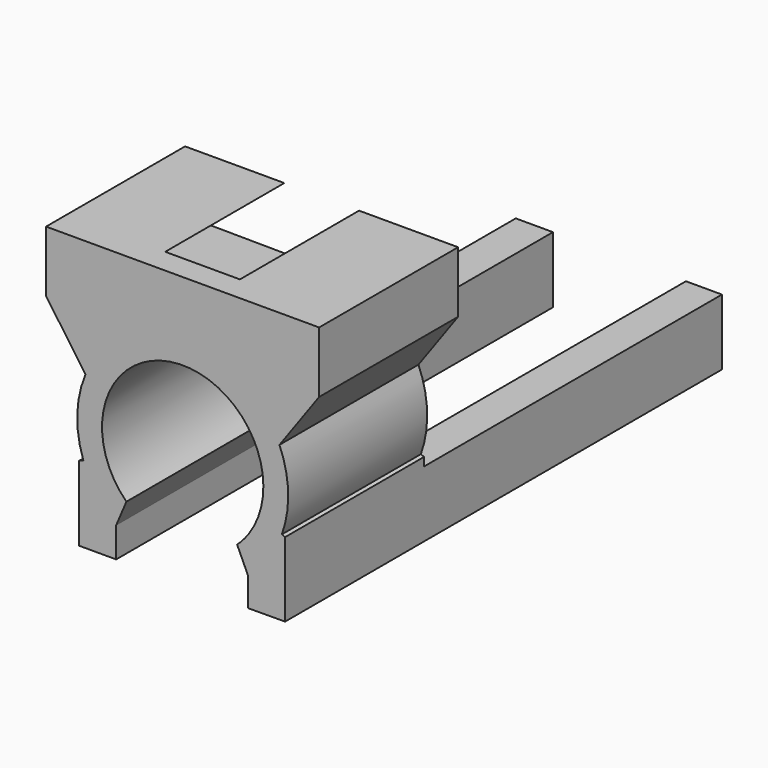
from build123d import *

# Parameters (mm, degrees)
F1_DEPTH = 7
F2_DEPTH = 6
F3_DEPTH = 15


# Not quite as in the source:
# - a feature names something its author has since deleted; it is built from what else it names


with BuildPart() as f1:
    # F0 (on Front) → F1 (new body)
    with BuildSketch(Plane.XZ):
        with BuildLine():
            Line((-3.9138396984, -1.8700768013), (-3.3236176952, -1.6008211246))
            Line((-3.3236176952, -1.6008211246), (-3.3236176952, -2.2903047641))
            Line((-3.3236176952, -2.2903047641), (-2.590710345, -2.2903047641))
            Line((-2.590710345, -2.2903047641), (-2.590710345, -3.7436034497))
            Line((-2.590710345, -3.7436034497), (-2.1779115118, -2.7734910012))
            ThreePointArc((-2.1779115118, -2.7734910012), (-0.2255882059, 2.7885019734), (2.7665772748, -2.2903047641))
            Line((2.7665772748, -2.2903047641), (3.4491920394, -2.2903047641))
            Line((3.4491920394, -2.2903047641), (3.4491920394, -1.6408955531))
            Line((3.4491920394, -1.6408955531), (4.0849162776, -1.8976975874))
            ThreePointArc((4.0849162776, -1.8976975874), (4.3385221106, -0.3163391945), (3.988877441, 1.2465935905))
            Line((3.988877441, 1.2465935905), (5.5865912817, 3.465253188))
            Line((5.5865912817, 3.465253188), (5.5865912817, 5.931237081))
            Line((5.5865912817, 5.931237081), (1.5955031972, 5.931237081))
            Line((1.5955031972, 5.931237081), (4.5903746292, 3.397220974))
            Line((4.5903746292, 3.397220974), (0.0905031972, 3.431237081))
            Line((0.0905031972, 3.431237081), (-4.4093682348, 3.465253188))
            Line((-4.4093682348, 3.465253188), (-1.4144968028, 5.931237081))
            Line((-1.4144968028, 5.931237081), (-5.4144968028, 5.931237081))
            Line((-5.4144968028, 5.931237081), (-5.4144968028, 3.465253188))
            Line((-5.4144968028, 3.465253188), (-3.8254308087, 1.2055638243))
            ThreePointArc((-3.8254308087, 1.2055638243), (-4.1577420716, -0.3239748955), (-3.9138396984, -1.8700768013))
        make_face()
        Polygon((-3.3236176952, -2.2903047641), (-3.3236176952, -1.6008211246), (-3.9138396984, -1.8700768013), (-4.090710345, -1.9507641112), (-4.090710345, -2.2903047641), align=None)
        Polygon((-2.590710345, -2.2903047641), (-3.3236176952, -2.2903047641), (-4.090710345, -2.2903047641), (-4.090710345, -4.9565606735), (-3.3236176952, -4.9565606735), (-2.590710345, -4.9565606735), (-2.590710345, -3.7436034497), align=None)
        with BuildLine():
            Line((3.4491920394, -2.2903047641), (2.7665772748, -2.2903047641))
            ThreePointArc((2.7665772748, -2.2903047641), (2.7416681899, -2.3259370036), (2.7162846892, -2.3612328517))
            Line((2.7162846892, -2.3612328517), (2.7162846892, -3.7879117456))
            Line((2.7162846892, -3.7879117456), (2.7162846892, -4.9565606735))
            Line((2.7162846892, -4.9565606735), (4.2162846892, -4.9497258588))
            Line((4.2162846892, -4.9497258588), (4.2162846892, -2.2903047641))
            Line((4.2162846892, -2.2903047641), (3.4491920394, -2.2903047641))
        make_face()
        with BuildLine():
            ThreePointArc((2.7162846892, -2.3612328517), (2.7416681899, -2.3259370036), (2.7665772748, -2.2903047641))
            Line((2.7665772748, -2.2903047641), (2.7162846892, -2.3612328517))
        make_face()
        Polygon((1.5955031972, 5.931237081), (-1.4144968028, 5.931237081), (-4.4093682348, 3.465253188), (0.0905031972, 3.431237081), (4.5903746292, 3.397220974), align=None)
        with BuildLine():
            Line((2.7162846892, -3.7879117456), (2.7162846892, -2.3612328517))
            ThreePointArc((2.7162846892, -2.3612328517), (2.5117247114, -2.6140814767), (2.2829176272, -2.8452189465))
            Line((2.2829176272, -2.8452189465), (2.7162846892, -3.7879117456))
        make_face()
        Polygon((3.4491920394, -1.6408955531), (3.4491920394, -2.2903047641), (4.2162846892, -2.2903047641), (4.2162846892, -1.9507641112), (4.0849162776, -1.8976975874), align=None)
    extrude(amount=F1_DEPTH)

    # F0 (on Front) → F2 (cut)
    with BuildSketch(Plane.XZ):
        Polygon((1.5955031972, 5.931237081), (-1.4144968028, 5.931237081), (-4.4093682348, 3.465253188), (0.0905031972, 3.431237081), (4.5903746292, 3.397220974), align=None)
    extrude(amount=F2_DEPTH, mode=Mode.SUBTRACT)

    # F0 (on Front) → F3 (join)
    with BuildSketch(Plane.XZ):
        Polygon((-2.590710345, -2.2903047641), (-3.3236176952, -2.2903047641), (-4.090710345, -2.2903047641), (-4.090710345, -4.9565606735), (-3.3236176952, -4.9565606735), (-2.590710345, -4.9565606735), (-2.590710345, -3.7436034497), align=None)
        with BuildLine():
            Line((3.4491920394, -2.2903047641), (2.7665772748, -2.2903047641))
            ThreePointArc((2.7665772748, -2.2903047641), (2.7416681899, -2.3259370036), (2.7162846892, -2.3612328517))
            Line((2.7162846892, -2.3612328517), (2.7162846892, -3.7879117456))
            Line((2.7162846892, -3.7879117456), (2.7162846892, -4.9565606735))
            Line((2.7162846892, -4.9565606735), (4.2162846892, -4.9497258588))
            Line((4.2162846892, -4.9497258588), (4.2162846892, -2.2903047641))
            Line((4.2162846892, -2.2903047641), (3.4491920394, -2.2903047641))
        make_face()
    extrude(amount=-F3_DEPTH)


solid = f1.part
